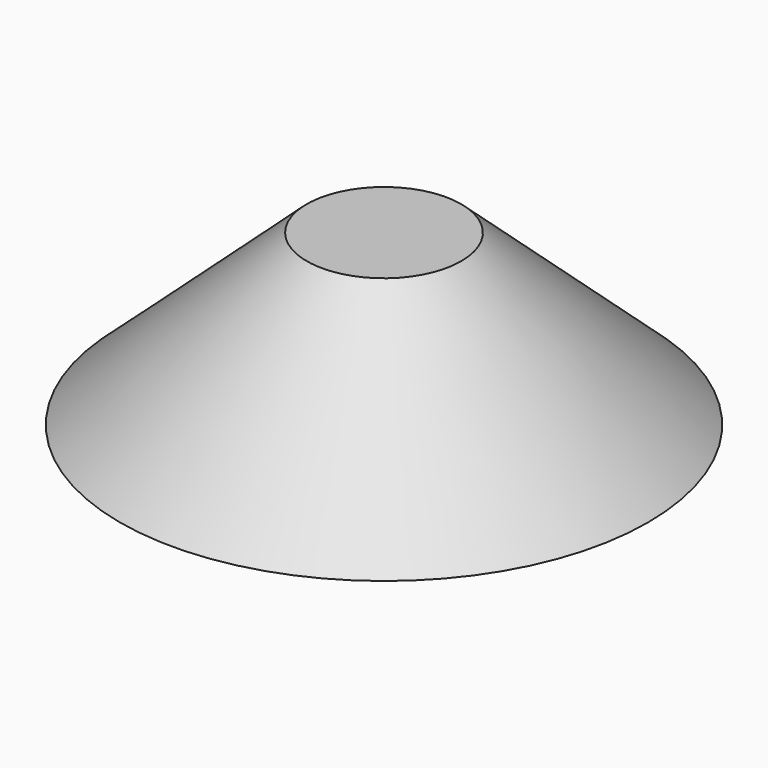
from build123d import *


# Not quite as in the source:
# - the program builds the solid bodies; features that only make, move or delete a surface that nothing else refers to are left out


with BuildPart() as f1:
    # F0 (on Front) → F1 (revolve)
    with BuildSketch(Plane.XZ):
        Polygon((41.9322475791, 0), (12.2643057257, 26.8646720797), (0, 26.8646720797), (0, 0), (12.4979112297, 0), align=None)
    revolve(axis=Axis((0, 0, 13.4323360398), (0, 0, -1)))


solid = f1.part
